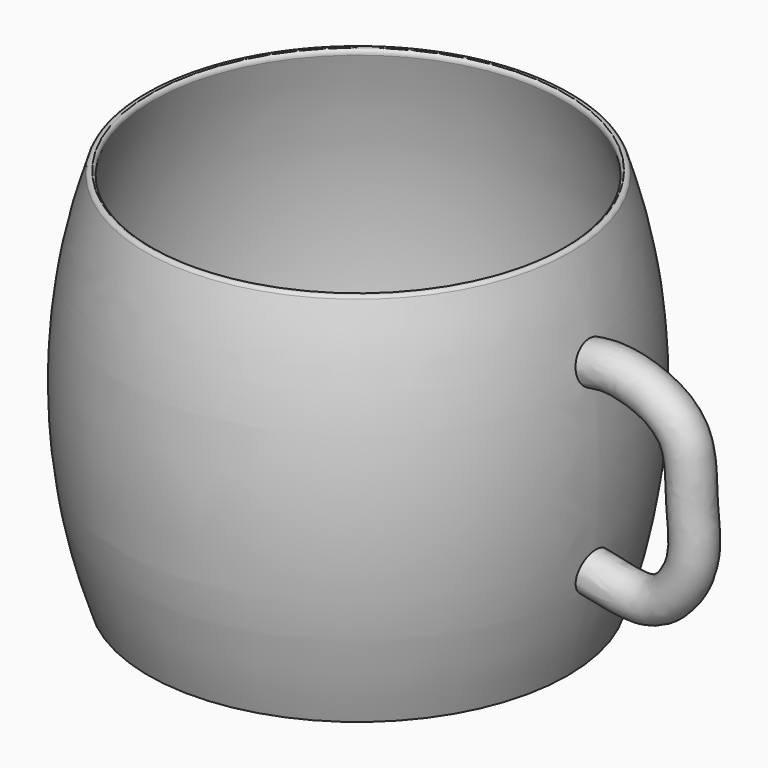
from build123d import *
from build123d import SkipClean  # not in build123d's __all__

# Parameters (mm, degrees)
F7_R      = 6.35
F9_DEPTH  = 0.508
F9_FACE_R = 6.35
F0_W      = 63.5
F0_H      = 2.54
F13_R     = 1.26999


# Not quite as in the source:
# - a fillet or chamfer is up to 0.001 mm smaller than in the source, because OpenCascade refuses the exact size


with BuildPart() as f9:
    # F7 (on line) → F9 (new body)
    with BuildSketch(Plane(origin=(82.6548274491, 0, 13.2568026813), x_dir=(0, 1, 0), z_dir=(0.987380869, 0, 0.1583635676))):
        with Locations((0, 75.5435333763)):
            Circle(F7_R)
    extrude(amount=F9_DEPTH)

    # F10: sweep along a path in F8
    with BuildLine(Plane.XZ) as f10_path:
        add(Plane.XZ * Edge.make_bspline(
            [(70.7532390952, 87.8850668669), (76.9328166344, 89.9386797191), (88.8710249029, 88.5008376395), (104.370995623, 79.193138841), (103.4524982391, 59.5380260798), (106.5599850718, 43.3373405944), (93.4955967823, 25.126711502), (79.9906905785, 29.9105676106), (71.9284340739, 31.3059575856)],
            knots=[0, 0, 0, 0, 0.1677820863, 0.3247840807, 0.4922297949, 0.6536282129, 0.8192284485, 1, 1, 1, 1], degree=3))
    # F9_face (on face) → F10 (sweep)
    with BuildSketch(Plane(origin=(71.1930734784, 0, 87.9274910061), x_dir=(0, 1, 0), z_dir=(0.987380869, 0, 0.1583635676))):
        Circle(F9_FACE_R)
    with SkipClean():  # cleaning this boolean's faces spoils the solid; the shape is the same uncleaned
        sweep(path=f10_path.line)

    # F1 (on Front) → F12 (revolve)
    with BuildSketch(Plane.XZ):
        with BuildLine():
            ThreePointArc((63.5, 116.84), (72.9351654888, 59.69), (63.5, 2.54))
            Line((63.5, 2.54), (63.5, 0))
            Line((63.5, 0), (65.3104266168, 0))
            ThreePointArc((65.3104266168, 0), (75.4728611683, 58.7783438109), (65.9052119216, 117.6564285714))
            Line((65.9052119216, 117.6564285714), (63.5, 116.84))
        make_face()
    revolve(axis=Axis((0, 0, 54.1628114879), (0, 0, 1)))

    # F13 (radius 1.27 in the source; OpenCascade refuses exactly that, so slightly less here)
    f13_edges = [f9.edges().sort_by_distance(p)[0] for p in [
        (-65.905212, 0, 117.656429),
        (-63.5, 0, 116.84),
    ]]
    fillet(f13_edges, radius=F13_R)


with BuildPart() as f11:
    # F0 (on Front) → F11 (revolve)
    with BuildSketch(Plane.XZ):
        with Locations((31.75, 1.27)):
            Rectangle(F0_W, F0_H)
    revolve(axis=Axis((0, 0, 54.1628114879), (0, 0, 1)))


solid = Compound([f9.part, f11.part])
